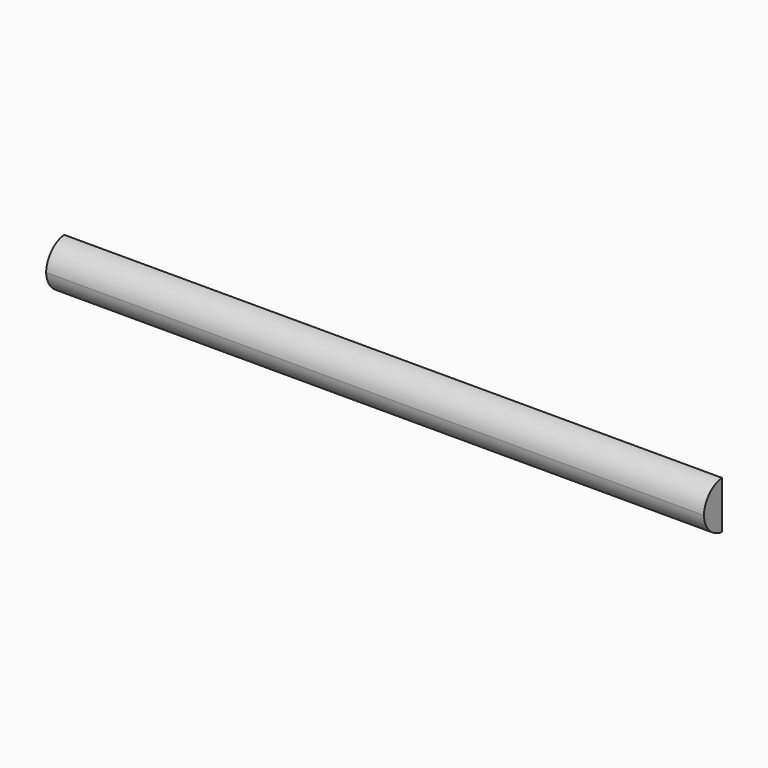
from build123d import *

# Parameters (mm, degrees)
F0_W        = 52.4768503383
F0_H        = 3.8066878915
F1_DEPTH    = 1.8
F2_T1_DEPTH = 62.4267247093


# Not quite as in the source:
# - a fillet or chamfer that OpenCascade refuses, or shapes differently, is made with other operations: its cross-section is extruded or revolved along the edge and cut away or added


with BuildPart() as f1:
    # F0 (on Front) → F1 (new body)
    with BuildSketch(Plane.XZ):
        with Locations((-16.5643407963, 30.3033739328)):
            Rectangle(F0_W, F0_H)
    extrude(amount=F1_DEPTH)

    # F2: fillet of radius 2 on 2 edges, made by hand

    # F2_s2 → F2_t1 (cut)
    with BuildSketch(Plane.YZ.offset(-47.777703151)):
        with BuildLine():
            ThreePointArc((0, 32.2067178786), (-1.2832396974, 31.5583837909), (-1.8, 30.2167430044))
            Line((-1.8, 30.2167430044), (-1.8, 32.2067178786))
            Line((-1.8, 32.2067178786), (0, 32.2067178786))
        make_face()
        with BuildLine():
            ThreePointArc((0, 28.4000299871), (-1.2832396974, 29.0483640748), (-1.8, 30.3900048613))
            Line((-1.8, 30.3900048613), (-1.8, 28.4000299871))
            Line((-1.8, 28.4000299871), (0, 28.4000299871))
        make_face()
    extrude(amount=F2_T1_DEPTH, mode=Mode.SUBTRACT)


solid = f1.part
